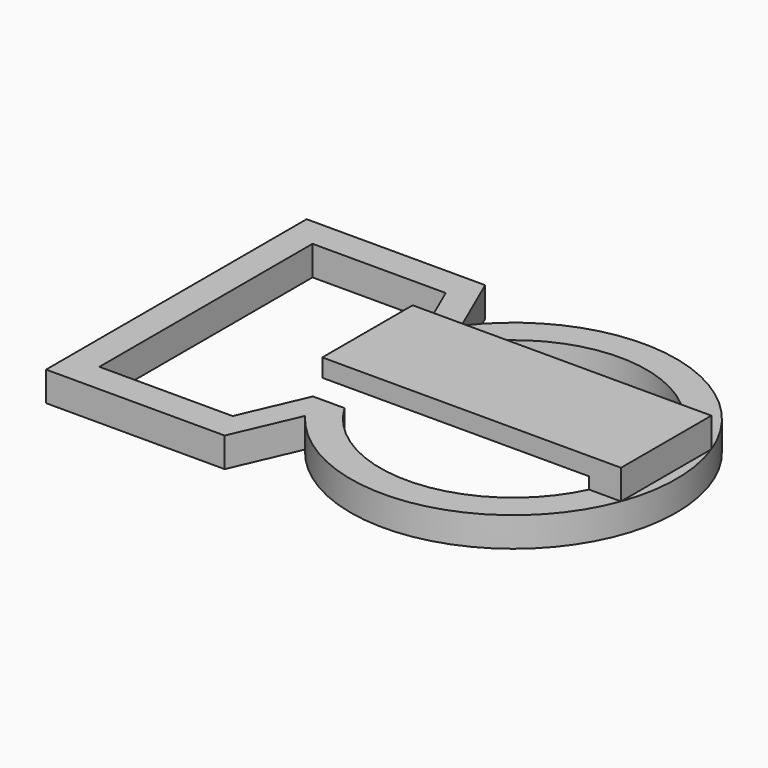
from build123d import *

# Parameters (mm, degrees)
F3_DEPTH = 12.7
F5_DEPTH = 12.7
F6_DEPTH = 5


# Not quite as in the source:
# - a feature names something its author has since deleted; it is built from what else it names


with BuildPart() as f3:
    # F2 (on Top) → F3 (new body)
    with BuildSketch(Plane.XY):
        with BuildLine():
            Line((-3.986357704, 43.8342139564), (-16.1254491208, 71.7667039931))
            Line((-16.1254491208, 71.7667039931), (-92.733014825, 71.7667039931))
            Line((-92.733014825, 71.7667039931), (-92.733014825, -67.9332960069))
            Line((-92.733014825, -67.9332960069), (-16.1254491208, -67.9332960069))
            Line((-16.1254491208, -67.9332960069), (-3.986357704, -40.0008059702))
            ThreePointArc((-3.986357704, -40.0008059702), (121.738009035, 1.9167039931), (-3.986357704, 43.8342139564))
        make_face()
        with BuildLine():
            Line((-80.033014825, -55.2332960069), (-80.033014825, 59.0667039931))
            Line((-80.033014825, 59.0667039931), (-22.883014825, 59.0667039931))
            Line((-22.883014825, 59.0667039931), (-10.7439288273, 31.1342139564))
            Line((-10.7439288273, 31.1342139564), (2.7712134193, 31.1342139564))
            ThreePointArc((2.7712134193, 31.1342139564), (109.038009035, 1.9167039931), (2.7712134193, -27.3008059702))
            Line((2.7712134193, -27.3008059702), (-10.7439288273, -27.3008059702))
            Line((-10.7439288273, -27.3008059702), (-22.883014825, -55.2332960069))
            Line((-22.883014825, -55.2332960069), (-80.033014825, -55.2332960069))
        make_face(mode=Mode.SUBTRACT)
    extrude(amount=F3_DEPTH)

    # F4 (on face) → F5 (join)
    with BuildSketch(Plane.XY.offset(12.7)):
        with BuildLine():
            Line((103.6531972523, 26.1342139564), (-10.7439288273, 26.1342139564))
            Line((-10.7439288273, 26.1342139564), (-10.7439288273, -22.3008059702))
            Line((-10.7439288273, -22.3008059702), (103.6531972523, -22.3008059702))
            ThreePointArc((103.6531972523, -22.3008059702), (109.038009035, 1.9167039931), (103.6531972523, 26.1342139564))
        make_face()
        with BuildLine():
            Line((117.405447257, 26.1342139564), (103.6531972523, 26.1342139564))
            ThreePointArc((103.6531972523, 26.1342139564), (109.038009035, 1.9167039931), (103.6531972523, -22.3008059702))
            Line((103.6531972523, -22.3008059702), (117.405447257, -22.3008059702))
            Line((117.405447257, -22.3008059702), (117.405447257, 26.1342139564))
        make_face()
    extrude(amount=F5_DEPTH)

    # F6 (cut): a face of the model
    f6_faces = [f3.faces().sort_by_distance(p)[0] for p in [
        (48.2779564243, 1.9167039931, 12.7),
    ]]
    extrude(f6_faces, amount=-F6_DEPTH, mode=Mode.SUBTRACT)


solid = f3.part
